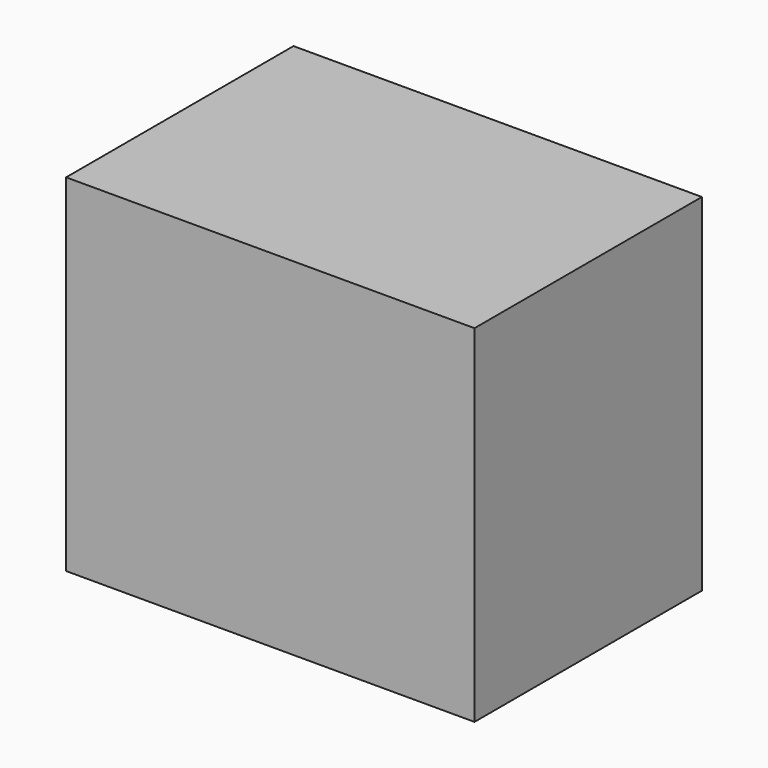
from build123d import *

# Parameters (mm, degrees)
F0_W     = 43.1057997048
F0_H     = 36.5860536695
F1_DEPTH = 30


# Not quite as in the source:
# - the program builds the solid bodies; features that only make, move or delete a surface that nothing else refers to are left out


with BuildPart() as f1:
    # F0 (on Front) → F1 (new body)
    with BuildSketch(Plane.XZ):
        with Locations((21.5528998524, 18.2930268347)):
            Rectangle(F0_W, F0_H)
    extrude(amount=-F1_DEPTH)


solid = f1.part
